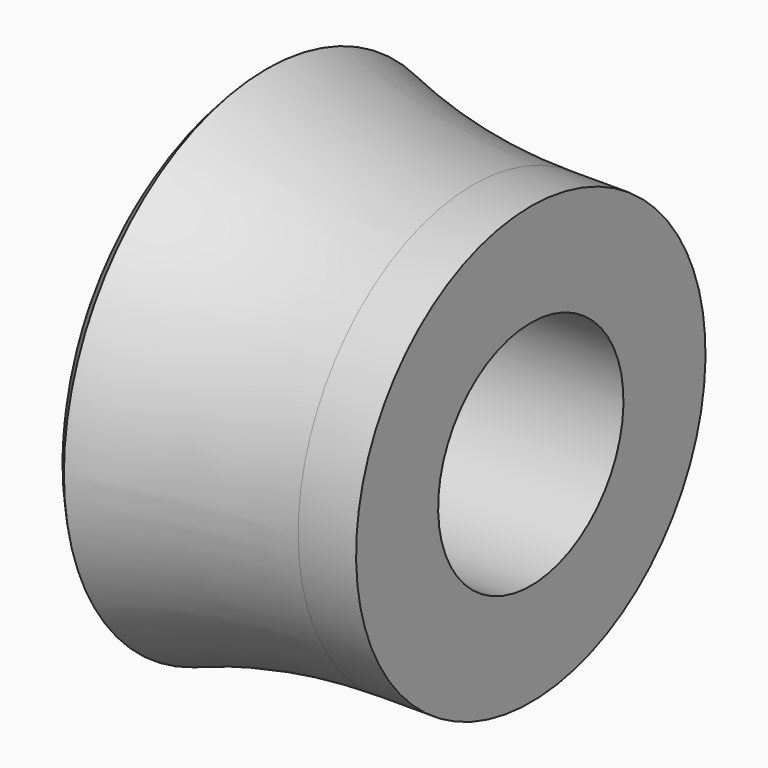
from build123d import *


# Not quite as in the source:
# - a fillet or chamfer that OpenCascade refuses, or shapes differently, is made with other operations: its cross-section is extruded or revolved along the edge and cut away or added


with BuildPart() as f1:
    # F0 (on Front) → F1 (revolve)
    with BuildSketch(Plane.XZ):
        with BuildLine():
            Line((0, 8.89), (0, 4.064))
            Line((0, 4.064), (10.795, 4.064))
            Line((10.795, 4.064), (10.795, 7.6631972609))
            Line((10.795, 7.6631972609), (8.763, 7.6631972609))
            ThreePointArc((8.763, 7.6631972609), (5.0918909727, 7.9720690296), (1.524, 8.89))
            Line((1.524, 8.89), (0, 8.89))
        make_face()
    revolve(axis=Axis((10.4300994426, 0, 0), (1, 0, 0)))

    # F2: fillet of radius 5.08 on 1 edges, made by hand

    # F2_s1 → F2_t2 (revolve, cut)
    with BuildSketch(Plane.XZ):
        with BuildLine():
            ThreePointArc((1.524, 8.89), (0.3964714157, 7.2296298982), (0, 5.2621543583))
            Line((0, 5.2621543583), (0, 8.89))
            Line((0, 8.89), (1.524, 8.89))
        make_face()
    revolve(axis=Axis((0, 0, 0), (1, 0, 0)), mode=Mode.SUBTRACT)


solid = f1.part
